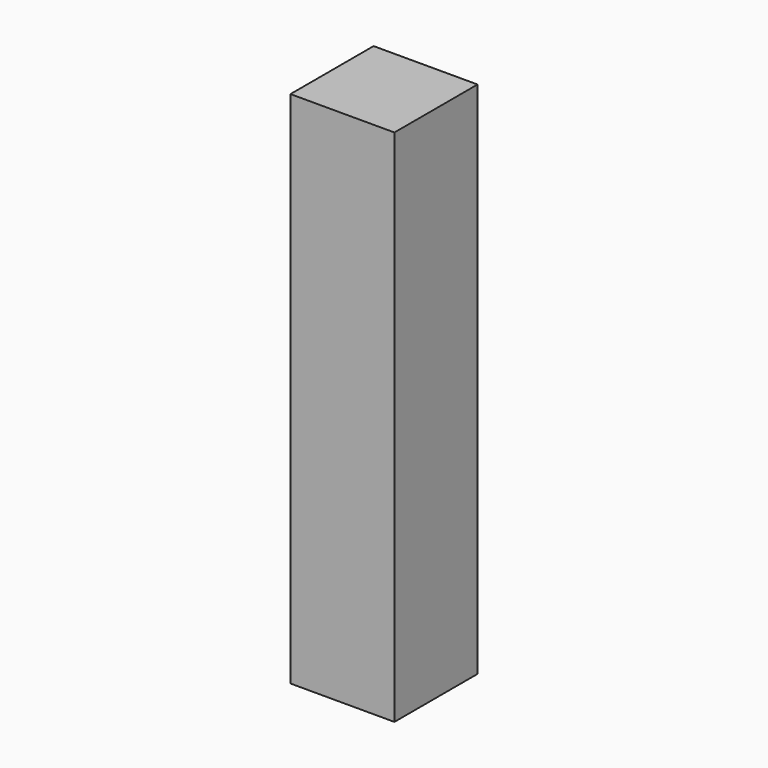
from build123d import *

# Parameters (mm, degrees)
F0_R     = 15
F1_DEPTH = 12.5
F2_W     = 10.0157754496
F2_H     = 10.012964718
F3_DEPTH = 25
F4_DEPTH = 25


# Not quite as in the source:
# - a feature of the source that left no trace in its solid (it failed there, or was rolled back) is left out


with BuildPart() as f1:
    # F0 (on Top) → F1 (new body, symmetric)
    with BuildSketch(Plane.XY):
        Circle(F0_R)
    extrude(amount=F1_DEPTH, both=True)

    # F2 (on face) → F3 (join)
    with BuildSketch(Plane.XY.offset(12.5)):
        Rectangle(F2_W, F2_H)
    extrude(amount=F3_DEPTH)

    # F4 (cut): a face of the model
    f4_faces = [f1.faces().sort_by_distance(p)[0] for p in [
        (-14.5757359313, 0, 12.5),
    ]]
    extrude(f4_faces, amount=-F4_DEPTH, mode=Mode.SUBTRACT)


solid = f1.part
